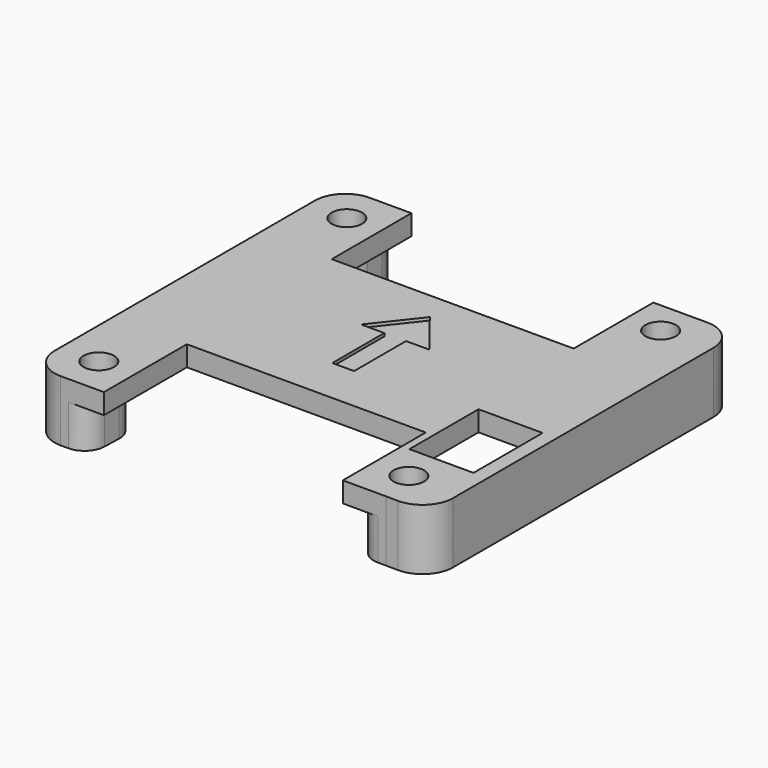
from build123d import *

# Parameters (mm, degrees)
F0_R         = 1.5
F1_DEPTH     = 2
F2_DEPTH     = 4
F3_T1_DEPTH  = 9
F4_T4_DEPTH  = 9
F4_T6_DEPTH  = 4
F4_T8_DEPTH  = 9
F4_T10_DEPTH = 8.8612846748
F4_T12_DEPTH = 9
F4_T14_DEPTH = 9
F5_R         = 3
F6_R         = 3
F8_DEPTH     = 0.3


# Not quite as in the source:
# - a fillet or chamfer that OpenCascade refuses, or shapes differently, is made with other operations: its cross-section is extruded or revolved along the edge and cut away or added


with BuildPart() as f1:
    # F0 (on Top) → F1 (new body)
    with BuildSketch(Plane.XY):
        with BuildLine():
            Line((11.75, -19), (13.2, -19))
            Line((13.2, -19), (13.2, -15.25))
            ThreePointArc((13.2, -15.25), (13.8004310986, -13.8004310986), (15.25, -13.2))
            Line((15.25, -13.2), (19, -13.2))
            Line((19, -13.2), (19, -11.75))
            Line((19, -11.75), (18.8090763986, -11.75))
            Line((18.8090763986, -11.75), (12.5, -11.75))
            Line((12.5, -11.75), (12.5, -3.25))
            Line((12.5, -3.25), (18.8090763986, -3.25))
            Line((18.8090763986, -3.25), (19, -3.25))
            Line((19, -3.25), (19, 13.6544716179))
            Line((19, 13.6544716179), (15.25, 13.6544716179))
            ThreePointArc((15.25, 13.6544716179), (13.8004310986, 14.2549027165), (13.2, 15.7044716179))
            Line((13.2, 15.7044716179), (13.2, 19))
            Line((13.2, 19), (11.9, 19))
            Line((11.9, 19), (11.9, 9.2))
            Line((11.9, 9.2), (0, 9.2))
            Line((0, 9.2), (-11.9, 9.2))
            Line((-11.9, 9.2), (-11.9, 19))
            Line((-11.9, 19), (-13.2, 19))
            Line((-13.2, 19), (-13.2, 15.25))
            ThreePointArc((-13.2, 15.25), (-13.8004310986, 13.8004310986), (-15.25, 13.2))
            Line((-15.25, 13.2), (-19, 13.2))
            Line((-19, 13.2), (-19, -13.2))
            Line((-19, -13.2), (-15.25, -13.2))
            ThreePointArc((-15.25, -13.2), (-13.7801859172, -13.8209630649), (-13.2008111101, -15.3076618908))
            Line((-13.2008111101, -15.3076618908), (-13.304709388, -19))
            Line((-13.304709388, -19), (-11.75, -19))
            Line((-11.75, -19), (-11.75, -8.8))
            Line((-11.75, -8.8), (11.75, -8.8))
            Line((11.75, -8.8), (11.75, -19))
        make_face()
        with BuildLine():
            Line((-19, 16), (-19, 13.2))
            Line((-19, 13.2), (-15.25, 13.2))
            ThreePointArc((-15.25, 13.2), (-13.8004310986, 13.8004310986), (-13.2, 15.25))
            Line((-13.2, 15.25), (-13.2, 19))
            Line((-13.2, 19), (-16, 19))
            ThreePointArc((-16, 19), (-18.1213203436, 18.1213203436), (-19, 16))
        make_face()
        with Locations((-15.25, 15.25)):
            Circle(F0_R, mode=Mode.SUBTRACT)
        with BuildLine():
            Line((13.2, -19), (16, -19))
            Line((16, -19), (20.2087182552, -19.0532333363))
            Line((20.2087182552, -19.0532333363), (20.2087182552, 18.9976152033))
            Line((20.2087182552, 18.9976152033), (16, 19))
            Line((16, 19), (13.2, 19))
            Line((13.2, 19), (13.2, 15.7044716179))
            ThreePointArc((13.2, 15.7044716179), (13.8004310986, 14.2549027165), (15.25, 13.6544716179))
            Line((15.25, 13.6544716179), (19, 13.6544716179))
            Line((19, 13.6544716179), (19, -3.25))
            Line((19, -3.25), (18.8090763986, -3.25))
            Line((18.8090763986, -3.25), (18.8090763986, -11.75))
            Line((18.8090763986, -11.75), (19, -11.75))
            Line((19, -11.75), (19, -13.2))
            Line((19, -13.2), (15.25, -13.2))
            ThreePointArc((15.25, -13.2), (13.8004310986, -13.8004310986), (13.2, -15.25))
            Line((13.2, -15.25), (13.2, -19))
        make_face()
        with Locations((15.25, -15.25)):
            Circle(F0_R, mode=Mode.SUBTRACT)
        with Locations((15.25, 15.7044716179)):
            Circle(F0_R, mode=Mode.SUBTRACT)
        with BuildLine():
            Line((-16, -19), (-13.304709388, -19))
            Line((-13.304709388, -19), (-13.2008111101, -15.3076618908))
            ThreePointArc((-13.2008111101, -15.3076618908), (-13.7801859172, -13.8209630649), (-15.25, -13.2))
            Line((-15.25, -13.2), (-19, -13.2))
            Line((-19, -13.2), (-19, -16))
            ThreePointArc((-19, -16), (-18.1213203436, -18.1213203436), (-16, -19))
        make_face()
        with Locations((-15.25, -15.25)):
            Circle(F0_R, mode=Mode.SUBTRACT)
    extrude(amount=F1_DEPTH)

    # F0 (on Top) → F2 (join)
    with BuildSketch(Plane.XY):
        with BuildLine():
            Line((-16, -19), (-13.304709388, -19))
            Line((-13.304709388, -19), (-13.2008111101, -15.3076618908))
            ThreePointArc((-13.2008111101, -15.3076618908), (-13.7801859172, -13.8209630649), (-15.25, -13.2))
            Line((-15.25, -13.2), (-19, -13.2))
            Line((-19, -13.2), (-19, -16))
            ThreePointArc((-19, -16), (-18.1213203436, -18.1213203436), (-16, -19))
        make_face()
        with Locations((-15.25, -15.25)):
            Circle(F0_R, mode=Mode.SUBTRACT)
        with BuildLine():
            Line((13.2, -19), (16, -19))
            Line((16, -19), (20.2087182552, -19.0532333363))
            Line((20.2087182552, -19.0532333363), (20.2087182552, 18.9976152033))
            Line((20.2087182552, 18.9976152033), (16, 19))
            Line((16, 19), (13.2, 19))
            Line((13.2, 19), (13.2, 15.7044716179))
            ThreePointArc((13.2, 15.7044716179), (13.8004310986, 14.2549027165), (15.25, 13.6544716179))
            Line((15.25, 13.6544716179), (19, 13.6544716179))
            Line((19, 13.6544716179), (19, -3.25))
            Line((19, -3.25), (18.8090763986, -3.25))
            Line((18.8090763986, -3.25), (18.8090763986, -11.75))
            Line((18.8090763986, -11.75), (19, -11.75))
            Line((19, -11.75), (19, -13.2))
            Line((19, -13.2), (15.25, -13.2))
            ThreePointArc((15.25, -13.2), (13.8004310986, -13.8004310986), (13.2, -15.25))
            Line((13.2, -15.25), (13.2, -19))
        make_face()
        with Locations((15.25, -15.25)):
            Circle(F0_R, mode=Mode.SUBTRACT)
        with Locations((15.25, 15.7044716179)):
            Circle(F0_R, mode=Mode.SUBTRACT)
        with BuildLine():
            Line((-19, 16), (-19, 13.2))
            Line((-19, 13.2), (-15.25, 13.2))
            ThreePointArc((-15.25, 13.2), (-13.8004310986, 13.8004310986), (-13.2, 15.25))
            Line((-13.2, 15.25), (-13.2, 19))
            Line((-13.2, 19), (-16, 19))
            ThreePointArc((-16, 19), (-18.1213203436, 18.1213203436), (-19, 16))
        make_face()
        with Locations((-15.25, 15.25)):
            Circle(F0_R, mode=Mode.SUBTRACT)
    extrude(amount=-F2_DEPTH)

    # F3: fillet of radius 2 on 1 edges, made by hand

    # F3_s2 → F3_t1 (cut)
    with BuildSketch(Plane.XY.offset(-9)):
        with BuildLine():
            ThreePointArc((-13.2, 17), (-13.7857864376, 18.4142135624), (-15.2, 19))
            Line((-15.2, 19), (-13.2, 19))
            Line((-13.2, 19), (-13.2, 17))
        make_face()
    extrude(amount=F3_T1_DEPTH, mode=Mode.SUBTRACT)

    # F4: fillet of radius 2 on 6 edges, made by hand


with BuildPart() as f4_tool2:
    # F4_s3 → F4_t4 (new body)
    with BuildSketch(Plane.XY.offset(5)):
        with BuildLine():
            ThreePointArc((17, 13.6544716179), (18.4142135624, 13.0686851803), (19, 11.6544716179))
            Line((19, 11.6544716179), (19, 13.6544716179))
            Line((19, 13.6544716179), (17, 13.6544716179))
        make_face()
    extrude(amount=-F4_T4_DEPTH)

    split(bisect_by=Plane.XY.offset(2), keep=Keep.BOTTOM)


with BuildPart() as f1_1:
    add(f1.part)

    # F4_t1: union F4_tool2
    add(f4_tool2.part)

    # F4_s7 → F4_t6 (join)
    with BuildSketch(Plane.XY.offset(-4)):
        with BuildLine():
            ThreePointArc((17.0771115477, -13.2), (18.2812710056, -12.7968719423), (19, -11.75))
            Line((19, -11.75), (19, -13.2))
            Line((19, -13.2), (17.0771115477, -13.2))
        make_face()
    extrude(amount=F4_T6_DEPTH)

    # F4_s9 → F4_t8 (cut)
    with BuildSketch(Plane.XY.offset(-9)):
        with BuildLine():
            ThreePointArc((-19, -15.2), (-18.4142135624, -13.7857864376), (-17, -13.2))
            Line((-17, -13.2), (-19, -13.2))
            Line((-19, -13.2), (-19, -15.2))
        make_face()
    extrude(amount=F4_T8_DEPTH, mode=Mode.SUBTRACT)

    # F4_s11 → F4_t10 (cut)
    with BuildSketch(Plane.XY.offset(-8.8612846748)):
        with BuildLine():
            ThreePointArc((-13.2500145849, -17.0562555032), (-13.8550408822, -18.4339649588), (-15.249223258, -19))
            Line((-15.249223258, -19), (-13.304709388, -19))
            Line((-13.304709388, -19), (-13.2500145849, -17.0562555032))
        make_face()
    extrude(amount=F4_T10_DEPTH, mode=Mode.SUBTRACT)

    # F4_s13 → F4_t12 (cut)
    with BuildSketch(Plane.XY.offset(-9)):
        with BuildLine():
            ThreePointArc((13.2, 17), (13.7857864376, 18.4142135624), (15.2, 19))
            Line((15.2, 19), (13.2, 19))
            Line((13.2, 19), (13.2, 17))
        make_face()
    extrude(amount=F4_T12_DEPTH, mode=Mode.SUBTRACT)

    # F4_s15 → F4_t14 (cut)
    with BuildSketch(Plane.XY.offset(-9)):
        with BuildLine():
            ThreePointArc((13.2, -17), (13.7857864376, -18.4142135624), (15.2, -19))
            Line((15.2, -19), (13.2, -19))
            Line((13.2, -19), (13.2, -17))
        make_face()
    extrude(amount=F4_T14_DEPTH, mode=Mode.SUBTRACT)

    # F5
    f5_edges = [f1_1.edges().sort_by_distance(p)[0] for p in [
        (20.208718, -19.053233, -1),
    ]]
    fillet(f5_edges, radius=F5_R)

    # F6
    f6_edges = [f1_1.edges().sort_by_distance(p)[0] for p in [
        (20.208718, 18.997615, -1),
    ]]
    fillet(f6_edges, radius=F6_R)

    # F7 (on face) → F8 (cut)
    with BuildSketch(Plane.XY.offset(2)):
        Polygon((-1.0717540281, -4.259434063), (1.0717540281, -4.259434063), (1.0717540281, 2.1297170315), (3.3500560094, 2.1297170315), (0, 6.3891510945), (-3.3500560094, 2.1297170315), (-1.0717540281, 2.1297170315), align=None)
    extrude(amount=-F8_DEPTH, mode=Mode.SUBTRACT)


solid = f1_1.part
